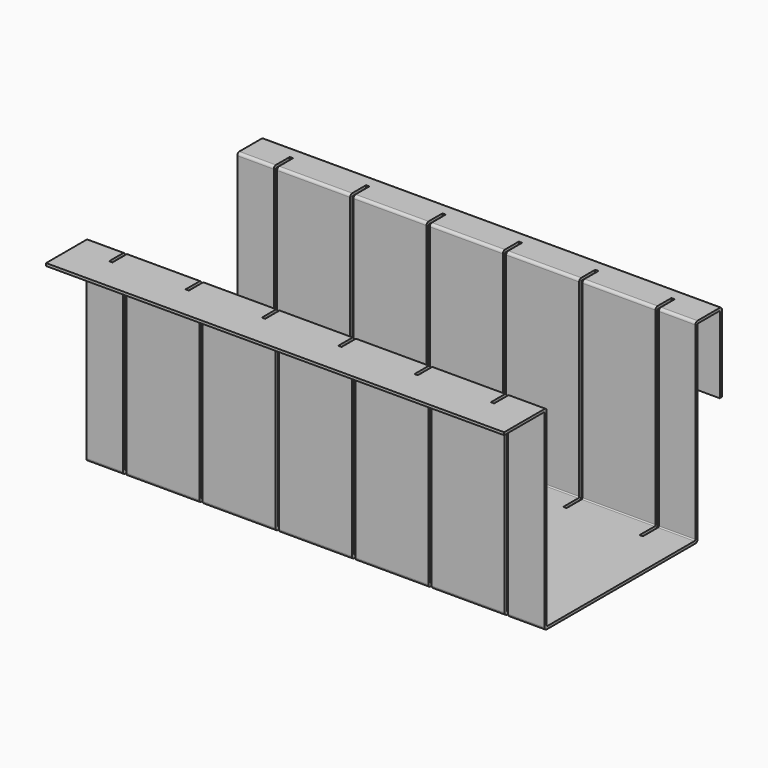
from build123d import *

# Parameters (mm, degrees)
F1_DEPTH  = 219.075
F2_W      = 1.5875
F2_H      = 19.0541078746
F3_DEPTH  = 97.282
F4_W      = 1.5875
F4_H      = 19.05
F5_DEPTH  = 93.346
F7_W      = 1.5875
F7_H      = 19.05
F8_DEPTH  = 134.62
F9_R      = 0.508
F10_R     = 1.27
F12_DEPTH = 8.128


with BuildPart() as f1:
    # F0 (on Right) → F1 (new body)
    with BuildSketch(Plane.YZ):
        Polygon((-37.2638233662, 38.1), (-62.6638233662, 38.1), (-62.6638233662, 36.83), (-38.5338233662, 36.83), (-38.5338233662, -55.245), (52.9061766338, -55.245), (52.9061766338, 36.83), (66.2411766338, 36.83), (66.2411766338, 0), (67.5111766338, 0), (67.5111766338, 38.1), (51.6361766338, 38.1), (51.6361766338, -53.975), (-37.2638233662, -53.975), align=None)
    extrude(amount=F1_DEPTH)

    # F2 (on face) → F3 (cut)
    with BuildSketch(Plane.XY.offset(38.1)):
        with Locations((18.25625, -37.2617694288)):
            Rectangle(F2_W, F2_H)
    extrude(amount=-F3_DEPTH, mode=Mode.SUBTRACT)

    # F4 (on face) → F5 (cut, through all)
    with BuildSketch(Plane.XY.offset(38.1)):
        with Locations((54.76875, -37.2638233662)):
            Rectangle(F4_W, F4_H)
        with Locations((91.28125, -37.2638233662)):
            Rectangle(F4_W, F4_H)
        with Locations((127.79375, -37.2638233662)):
            Rectangle(F4_W, F4_H)
        with Locations((164.30625, -37.2638233662)):
            Rectangle(F4_W, F4_H)
        with Locations((200.81875, -37.2638233662)):
            Rectangle(F4_W, F4_H)
    extrude(amount=-F5_DEPTH, mode=Mode.SUBTRACT)

    # F7 (on face) → F8 (cut)
    with BuildSketch(Plane.XY.offset(38.1)):
        with Locations((18.25625, 51.6361766338)):
            Rectangle(F7_W, F7_H)
        with Locations((54.76875, 51.6361766338)):
            Rectangle(F7_W, F7_H)
        with Locations((91.28125, 51.6361766338)):
            Rectangle(F7_W, F7_H)
        with Locations((127.79375, 51.6361766338)):
            Rectangle(F7_W, F7_H)
        with Locations((164.30625, 51.6361766338)):
            Rectangle(F7_W, F7_H)
        with Locations((200.81875, 51.6361766338)):
            Rectangle(F7_W, F7_H)
    extrude(amount=-F8_DEPTH, mode=Mode.SUBTRACT)

    # F9
    f9_edges = [f1.edges().sort_by_distance(p)[0] for p in [
        (182.5625, -38.533823, 36.83),
        (146.05, -38.533823, 36.83),
        (109.5375, -38.533823, 36.83),
        (73.025, -38.533823, 36.83),
        (36.5125, -38.533823, 36.83),
        (8.73125, -38.533823, 36.83),
        (182.5625, -37.263823, -53.975),
        (146.05, -37.263823, -53.975),
        (109.5375, -37.263823, -53.975),
        (73.025, -37.263823, -53.975),
        (36.5125, -37.263823, -53.975),
        (8.73125, -37.263823, -53.975),
        (210.34375, -37.263823, -53.975),
        (210.34375, -38.533823, 36.83),
        (8.73125, 52.906177, 36.83),
        (109.5375, 66.241177, 36.83),
        (210.34375, 52.906177, 36.83),
        (182.5625, 52.906177, 36.83),
        (146.05, 52.906177, 36.83),
        (109.5375, 52.906177, 36.83),
        (73.025, 52.906177, 36.83),
        (36.5125, 52.906177, 36.83),
        (8.73125, 51.636177, -53.975),
        (210.34375, 51.636177, -53.975),
        (182.5625, 51.636177, -53.975),
        (146.05, 51.636177, -53.975),
        (109.5375, 51.636177, -53.975),
        (73.025, 51.636177, -53.975),
        (36.5125, 51.636177, -53.975),
    ]]
    fillet(f9_edges, radius=F9_R)

    # F10
    f10_edges = [f1.edges().sort_by_distance(p)[0] for p in [
        (182.5625, -37.263823, 38.1),
        (146.05, -37.263823, 38.1),
        (109.5375, -37.263823, 38.1),
        (73.025, -37.263823, 38.1),
        (36.5125, -37.263823, 38.1),
        (8.73125, -37.263823, 38.1),
        (8.73125, -38.533823, -55.245),
        (36.5125, -38.533823, -55.245),
        (73.025, -38.533823, -55.245),
        (109.5375, -38.533823, -55.245),
        (146.05, -38.533823, -55.245),
        (182.5625, -38.533823, -55.245),
        (210.34375, -37.263823, 38.1),
        (8.73125, 52.906177, -55.245),
        (36.5125, 52.906177, -55.245),
        (73.025, 52.906177, -55.245),
        (109.5375, 52.906177, -55.245),
        (146.05, 52.906177, -55.245),
        (182.5625, 52.906177, -55.245),
        (210.34375, 52.906177, -55.245),
        (210.34375, -38.533823, -55.245),
        (8.73125, 51.636177, 38.1),
        (36.5125, 51.636177, 38.1),
        (73.025, 51.636177, 38.1),
        (109.5375, 51.636177, 38.1),
        (146.05, 51.636177, 38.1),
        (182.5625, 51.636177, 38.1),
        (210.34375, 51.636177, 38.1),
        (109.5375, 67.511177, 38.1),
    ]]
    fillet(f10_edges, radius=F10_R)

    # F11 (on face) → F12 (cut)
    with BuildSketch(Plane(origin=(0, 67.5111766338, 0), x_dir=(-1, 0, 0), z_dir=(0, 1, 0))):
        with BuildLine():
            Line((-180.18125, 15.5544459855), (-180.18125, 27.305))
            ThreePointArc((-180.18125, 27.305), (-182.5625, 29.68625), (-184.94375, 27.305))
            Line((-184.94375, 27.305), (-184.94375, 15.5544459855))
            ThreePointArc((-184.94375, 15.5544459855), (-182.5625, 6.6675), (-180.18125, 15.5544459855))
        make_face()
        with BuildLine():
            Line((-34.13125, 15.5544459855), (-34.13125, 27.305))
            ThreePointArc((-34.13125, 27.305), (-36.5125, 29.68625), (-38.89375, 27.305))
            Line((-38.89375, 27.305), (-38.89375, 15.5544459855))
            ThreePointArc((-38.89375, 15.5544459855), (-36.5125, 6.6675), (-34.13125, 15.5544459855))
        make_face()
    extrude(amount=-F12_DEPTH, mode=Mode.SUBTRACT)


solid = f1.part
